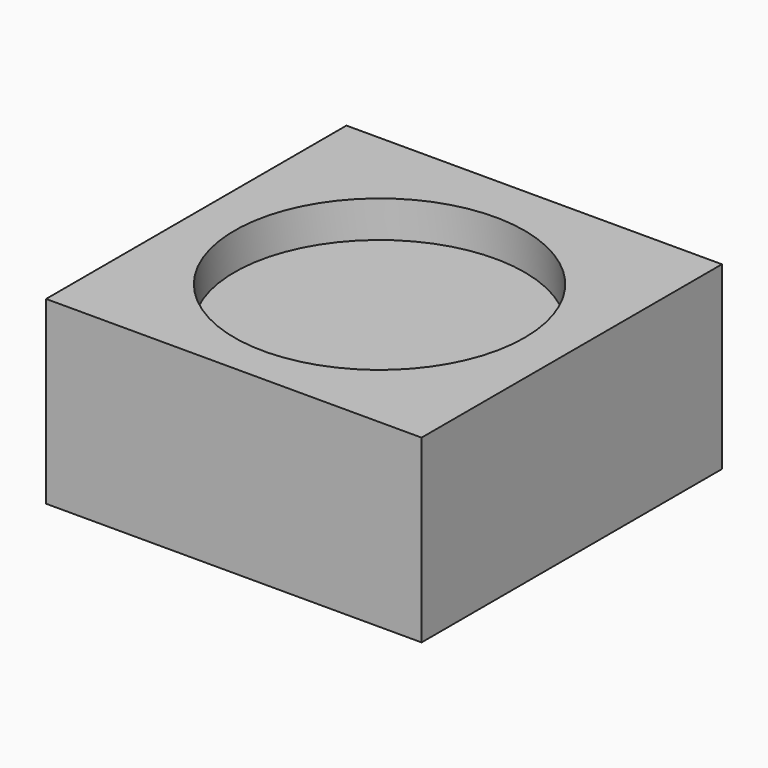
from build123d import *

# Parameters (mm, degrees)
F1_R     = 13.9916710172
F2_DEPTH = 25.4
F4_W     = 36.2210944295
F4_H     = 17.3936840147
F5_DEPTH = 36.2169072032
F6_DEPTH = 11.5376953036


with BuildPart() as f2:
    # F1 (on face) → F2 (new body)
    with BuildSketch(Plane.XY):
        Circle(F1_R)
    extrude(amount=F2_DEPTH)

    # F4 (on face) → F5 (join)
    with BuildSketch(Plane(origin=(0, -17.5722502172, 0), x_dir=(-1, 0, 0), z_dir=(0, 1, 0))):
        with Locations((0, 8.6968420073)):
            Rectangle(F4_W, F4_H)
    extrude(amount=F5_DEPTH)

    # F6 (cut): a face of the model
    f6_faces = [f2.faces().sort_by_distance(p)[0] for p in [
        (0, 0, 25.4),
    ]]
    extrude(f6_faces, amount=-F6_DEPTH, mode=Mode.SUBTRACT)


solid = f2.part
